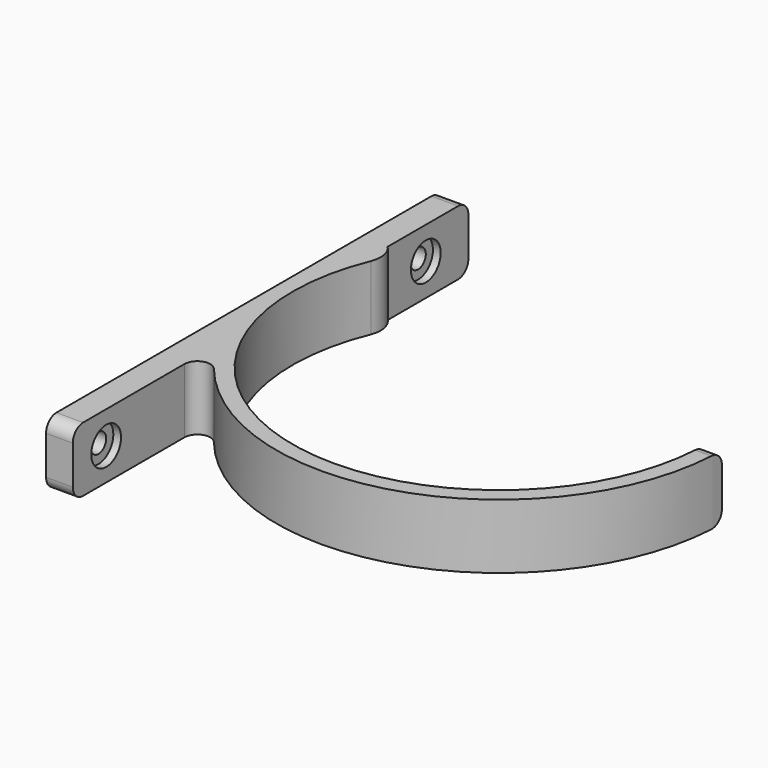
from build123d import *

# Parameters (mm, degrees)
F1_DEPTH    = 6.35
F2_R        = 2.54
F3_R        = 1.905
F4_DEPTH    = 25.4
F5_R        = 3.6608290009
F6_DEPTH    = 1.524
F7_T1_DEPTH = 34.0803226462


# Not quite as in the source:
# - a fillet or chamfer that OpenCascade refuses, or shapes differently, is made with other operations: its cross-section is extruded or revolved along the edge and cut away or added
# - a feature names something its author has since deleted; it is built from what else it names


with BuildPart() as f1:
    # F0 (on Top) → F1 (new body, symmetric)
    with BuildSketch(Plane.XY):
        with BuildLine():
            ThreePointArc((40.64, 0), (-9.9515149654, -39.402753075), (-35.7663459593, 19.2971007335))
            Line((-35.7663459593, 19.2971007335), (-38.5605917374, 20.8046867283))
            Line((-38.5605917374, 20.8046867283), (-38.5605917374, 40.64))
            Line((-38.5605917374, 40.64), (-43.815, 40.64))
            Line((-43.815, 40.64), (-43.815, -43.815))
            Line((-43.815, -43.815), (-43.815, -56.6207952306))
            Line((-43.815, -56.6207952306), (-38.5605917374, -56.6207952306))
            Line((-38.5605917374, -56.6207952306), (-38.5605917374, -43.815))
            Line((-38.5605917374, -43.815), (-38.5605917374, -20.8046867283))
            ThreePointArc((-38.5605917374, -20.8046867283), (10.7289770721, -42.481093159), (43.815, 0))
            Line((43.815, 0), (40.64, 0))
        make_face()
    extrude(amount=F1_DEPTH, both=True)

    # F2
    f2_edges = [f1.edges().sort_by_distance(p)[0] for p in [
        (42.2275, 0, 6.35),
        (42.2275, 0, -6.35),
        (-38.560592, -20.804687, 0),
        (-41.187796, 40.64, 6.35),
        (-41.187796, 40.64, -6.35),
        (-41.187796, -56.620795, 6.35),
        (-41.187796, -56.620795, -6.35),
    ]]
    fillet(f2_edges, radius=F2_R)

    # F3 (on face) → F4 (cut)
    with BuildSketch(Plane(origin=(-43.815, 0, 0), x_dir=(0, -1, 0), z_dir=(-1, 0, 0))):
        with Locations((-30.1695157966, 0)):
            Circle(F3_R)
        with Locations((48.4138801694, 0)):
            Circle(F3_R)
    extrude(amount=-F4_DEPTH, mode=Mode.SUBTRACT)

    # F5 (on face) → F6 (cut)
    with BuildSketch(Plane.YZ.offset(-38.5605917374)):
        with Locations((30.1695157966, 0)):
            Circle(F5_R)
        with Locations((-48.4138801694, 0)):
            Circle(F5_R)
    extrude(amount=-F6_DEPTH, mode=Mode.SUBTRACT)

    # F7: fillet of radius 5.08 on 1 edges, made by hand

    # F7_s2 → F7_t1 (cut)
    with BuildSketch(Plane.XY.offset(-17.0401613231)):
        with BuildLine():
            ThreePointArc((-37.5959569593, 15.4322266804), (-37.2954100255, 18.259021389), (-38.5605917374, 20.8046867283))
            Line((-38.5605917374, 20.8046867283), (-35.7663459593, 19.2971007335))
            ThreePointArc((-35.7663459593, 19.2971007335), (-36.7320185294, 17.3887439097), (-37.5959569593, 15.4322266804))
        make_face()
    extrude(amount=F7_T1_DEPTH, mode=Mode.SUBTRACT)


solid = f1.part
